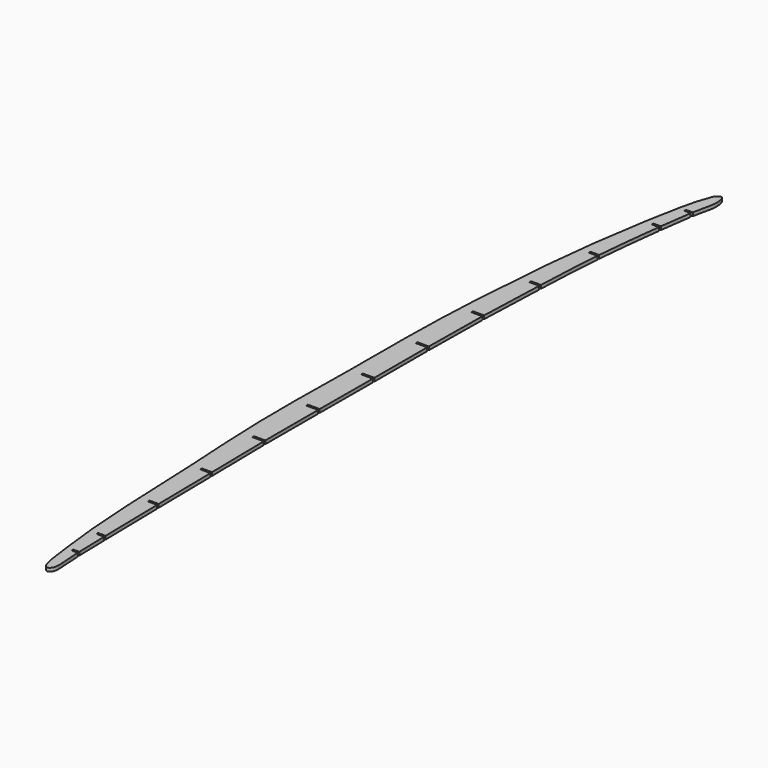
from build123d import *

# Parameters (mm, degrees)
F1_DEPTH = 10


# Not quite as in the source:
# - a feature names something its author has since deleted; it is built from what else it names


with BuildPart() as f1:
    # F0 (on Top) → F1 (new body)
    with BuildSketch(Plane.XY):
        with BuildLine():
            Line((-9.2522319783, 1105.5465694817), (-9.2522319783, 1108.5465694817))
            Line((-9.2522319783, 1108.5465694817), (-28.2522319783, 1108.5465694817))
            add(Edge.make_bspline(
                [(-28.2522319783, 1108.5465694817), (-34.1692287273, 1078.3481872981), (-40.0862254764, 1048.1498051145), (-46.885506853, 1008.5465694817)],
                knots=[0, 0, 0, 0, 0.0623728759, 0.0623728759, 0.0623728759, 0.0623728759], degree=3))
            Line((-46.885506853, 1008.5465694817), (-25.3817387583, 1008.5465694817))
            Line((-25.3817387583, 1008.5465694817), (-25.3817387583, 1011.5465694817))
            Line((-25.3817387583, 1011.5465694817), (-3.4951998214, 1011.5465694817))
            add(Edge.make_bspline(
                [(9.3214260817, 1105.5465694817), (5.2778951966, 1077.0910022719), (1.2125502532, 1048.3609188135), (-3.4951998214, 1011.5465694817)],
                knots=[0.0020582204, 0.0020582204, 0.0020582204, 0.0020582204, 0.0606128099, 0.0606128099, 0.0606128099, 0.0606128099], degree=3))
            Line((9.3214260817, 1105.5465694817), (-9.2522319783, 1105.5465694817))
        make_face()
        with BuildLine():
            Line((-28.2522319783, 1108.5465694817), (-9.2522319783, 1108.5465694817))
            Line((-9.2522319783, 1108.5465694817), (-9.2522319783, 1111.5465694817))
            Line((-9.2522319783, 1111.5465694817), (10.4483753261, 1111.5465694817))
            add(Edge.make_bspline(
                [(10.4483753261, 1111.5465694817), (14.2237569857, 1127.7176279013), (20.7843357368, 1156.0283342705), (24.50141426, 1181.1497468298), (21.913351831, 1202.3721726285), (17.2535020339, 1211.7645420112), (14.0231014783, 1212.5065694817)],
                knots=[0.0100141442, 0.0100141442, 0.0100141442, 0.0100141442, 0.1720322765, 0.2970501568, 0.4103591472, 0.4934759383, 0.4934759383, 0.4934759383, 0.4934759383], degree=3))
            add(Edge.make_bspline(
                [(14.0231014783, 1212.5065694817), (10.6916463361, 1213.2718093304), (0.9849483202, 1207.717065294), (-4.4652508998, 1194.4970040922), (-17.4495437423, 1158.8703779353), (-24.4328369098, 1126.3390394336), (-28.2522319783, 1108.5465694817)],
                knots=[0.4934759383, 0.4934759383, 0.4934759383, 0.4934759383, 0.5791928197, 0.6716390479, 0.8204084848, 1, 1, 1, 1], degree=3))
        make_face()
        with BuildLine():
            Line((-25.3817387583, 1008.5465694817), (-46.885506853, 1008.5465694817))
            add(Edge.make_bspline(
                [(-46.885506853, 1008.5465694817), (-56.4704307745, 952.7180223817), (-67.8086700034, 878.1997316325), (-76.2546409025, 808.5465694817)],
                knots=[0.0623728759, 0.0623728759, 0.0623728759, 0.0623728759, 0.1502997077, 0.1502997077, 0.1502997077, 0.1502997077], degree=3))
            Line((-76.2546409025, 808.5465694817), (-50.7523337375, 808.5465694817))
            Line((-50.7523337375, 808.5465694817), (-50.7523337375, 811.5465694817))
            Line((-50.7523337375, 811.5465694817), (-25.0042987138, 811.5465694817))
            add(Edge.make_bspline(
                [(-4.2590252459, 1005.5465694817), (-11.1919357354, 950.8419950912), (-19.4396527515, 879.0589079331), (-25.0042987138, 811.5465694817)],
                knots=[0.0637563334, 0.0637563334, 0.0637563334, 0.0637563334, 0.1487347177, 0.1487347177, 0.1487347177, 0.1487347177], degree=3))
            Line((-4.2590252459, 1005.5465694817), (-25.3817387583, 1005.5465694817))
            Line((-25.3817387583, 1005.5465694817), (-25.3817387583, 1008.5465694817))
        make_face()
        with BuildLine():
            Line((-50.7523337375, 808.5465694817), (-76.2546409025, 808.5465694817))
            add(Edge.make_bspline(
                [(-76.2546409025, 808.5465694817), (-84.6749646264, 739.1049172777), (-90.2205587707, 674.4988914733), (-95.4501271993, 608.5465694817)],
                knots=[0.1502997077, 0.1502997077, 0.1502997077, 0.1502997077, 0.2379595395, 0.2379595395, 0.2379595395, 0.2379595395], degree=3))
            Line((-95.4501271993, 608.5465694817), (-65.9492915816, 608.5465694817))
            Line((-65.9492915816, 608.5465694817), (-65.9492915816, 611.5465694817))
            Line((-65.9492915816, 611.5465694817), (-36.3208296657, 611.5465694817))
            add(Edge.make_bspline(
                [(-25.492600007, 805.5470480317), (-30.8991386303, 738.261256599), (-33.600522451, 675.484027067), (-36.3208296657, 611.5465694817)],
                knots=[0.1512568673, 0.1512568673, 0.1512568673, 0.1512568673, 0.2362855612, 0.2362855612, 0.2362855612, 0.2362855612], degree=3))
            Line((-25.492600007, 805.5470480317), (-50.8059161147, 805.5470480317))
            Line((-50.8059161147, 805.5470480317), (-50.7523337375, 808.5465694817))
        make_face()
        with BuildLine():
            Line((-65.9492915816, 608.5465694817), (-95.4501271993, 608.5465694817))
            add(Edge.make_bspline(
                [(-95.4501271993, 608.5465694817), (-100.6735657013, 542.6715546134), (-105.5817189232, 475.4533978756), (-108.8488180837, 408.5465694817)],
                knots=[0.2379595395, 0.2379595395, 0.2379595395, 0.2379595395, 0.3255166193, 0.3255166193, 0.3255166193, 0.3255166193], degree=3))
            Line((-108.8488180837, 408.5465694817), (-76.3366638949, 408.5465694817))
            Line((-76.3366638949, 408.5465694817), (-76.3366638949, 411.5465694817))
            Line((-76.3366638949, 411.5465694817), (-43.7472965242, 411.5465694817))
            add(Edge.make_bspline(
                [(-36.576081022, 605.5465694817), (-39.2965672487, 541.5968769288), (-42.0608997966, 476.4245488132), (-43.7472965243, 411.5465694817)],
                knots=[0.2389437345, 0.2389437345, 0.2389437345, 0.2389437345, 0.3238872962, 0.3238872962, 0.3238872962, 0.3238872962], degree=3))
            Line((-36.576081022, 605.5465694817), (-65.9492915816, 605.5465694817))
            Line((-65.9492915816, 605.5465694817), (-65.9492915816, 608.5465694817))
        make_face()
        with BuildLine():
            Line((-76.3366638949, 408.5465694817), (-108.8488180837, 408.5465694817))
            add(Edge.make_bspline(
                [(-108.8488180837, 408.5465694817), (-112.112873039, 341.7020832768), (-113.7389306982, 275.1683455095), (-114.3242902488, 208.5465694817)],
                knots=[0.3255166193, 0.3255166193, 0.3255166193, 0.3255166193, 0.4129921155, 0.4129921155, 0.4129921155, 0.4129921155], degree=3))
            Line((-114.3242902488, 208.5465694817), (-80.310060953, 208.5465694817))
            Line((-80.310060953, 208.5465694817), (-80.310060953, 211.5465694817))
            Line((-80.310060953, 211.5465694817), (-46.2853714025, 211.5465694817))
            add(Edge.make_bspline(
                [(-43.9001795453, 405.5465694817), (-45.519256644, 340.6971675299), (-46.0554016999, 276.1594412286), (-46.2853714025, 211.5465694817)],
                knots=[0.3265062426, 0.3265062426, 0.3265062426, 0.3265062426, 0.4114374445, 0.4114374445, 0.4114374445, 0.4114374445], degree=3))
            Line((-43.9001795453, 405.5465694817), (-76.3366638949, 405.5465694817))
            Line((-76.3366638949, 405.5465694817), (-76.3366638949, 408.5465694817))
        make_face()
        with BuildLine():
            Line((-80.310060953, 208.5465694817), (-114.3242902488, 208.5465694817))
            add(Edge.make_bspline(
                [(-114.3242902488, 208.5465694817), (-114.9095417049, 141.9370960513), (-114.4544793743, 75.2396168723), (-114.9729122534, 8.5465694817)],
                knots=[0.4129921155, 0.4129921155, 0.4129921155, 0.4129921155, 0.5004514582, 0.5004514582, 0.5004514582, 0.5004514582], degree=3))
            Line((-114.9729122534, 8.5465694817), (-80.772249135, 8.5465694817))
            Line((-80.772249135, 8.5465694817), (-80.772249135, 11.5465694817))
            Line((-80.772249135, 11.5465694817), (-46.5657327214, 11.5465694817))
            add(Edge.make_bspline(
                [(-46.3058677148, 205.5465694817), (-46.517541999, 140.9336478574), (-46.4426078998, 76.2408210046), (-46.5657327214, 11.5465694817)],
                knots=[0.4140662707, 0.4140662707, 0.4140662707, 0.4140662707, 0.4989910833, 0.4989910833, 0.4989910833, 0.4989910833], degree=3))
            Line((-46.3058677148, 205.5465694817), (-80.310060953, 205.5465694817))
            Line((-80.310060953, 205.5465694817), (-80.310060953, 208.5465694817))
        make_face()
        with BuildLine():
            Line((-80.772249135, 8.5465694817), (-114.9729122534, 8.5465694817))
            add(Edge.make_bspline(
                [(-114.9729122534, 8.5465694817), (-115.4913633728, -58.1488243975), (-116.9833782047, -124.8397861765), (-117.4326707445, -191.4534305183)],
                knots=[0.5004514582, 0.5004514582, 0.5004514582, 0.5004514582, 0.587913878, 0.587913878, 0.587913878, 0.587913878], degree=3))
            Line((-117.4326707445, -191.4534305183), (-82.4265356335, -191.4534305183))
            Line((-82.4265356335, -191.4534305183), (-82.4265356335, -188.4534305183))
            Line((-82.4265356335, -188.4534305183), (-47.4040323866, -188.4534305183))
            add(Edge.make_bspline(
                [(-46.5777314963, 5.5465694817), (-46.7134050172, -59.1479448978), (-47.0517150176, -123.8414273541), (-47.4040323866, -188.4534305183)],
                knots=[0.5016165032, 0.5016165032, 0.5016165032, 0.5016165032, 0.5865416442, 0.5865416442, 0.5865416442, 0.5865416442], degree=3))
            Line((-46.5777314963, 5.5465694817), (-80.772249135, 5.5465694817))
            Line((-80.772249135, 5.5465694817), (-80.772249135, 8.5465694817))
        make_face()
        with BuildLine():
            Line((-82.4265356335, -191.4534305183), (-117.4326707445, -191.4534305183))
            add(Edge.make_bspline(
                [(-117.4326707445, -191.4534305183), (-117.8819688578, -258.0679012195), (-117.2885188084, -324.6050525653), (-114.5979590791, -391.4534305183)],
                knots=[0.587913878, 0.587913878, 0.587913878, 0.587913878, 0.6753773828, 0.6753773828, 0.6753773828, 0.6753773828], degree=3))
            Line((-114.5979590791, -391.4534305183), (-81.0956338475, -391.4534305183))
            Line((-81.0956338475, -391.4534305183), (-81.0956338475, -388.4534305183))
            Line((-81.0956338475, -388.4534305183), (-47.6180785507, -388.4534305183))
            add(Edge.make_bspline(
                [(-47.4367827083, -194.4534305183), (-47.7896354912, -259.0626621028), (-48.1401096643, -323.5953829529), (-47.6180785507, -388.4534305183)],
                knots=[0.58917052, 0.58917052, 0.58917052, 0.58917052, 0.6740985981, 0.6740985981, 0.6740985981, 0.6740985981], degree=3))
            Line((-47.4367827083, -194.4534305183), (-82.4265356335, -194.4534305183))
            Line((-82.4265356335, -194.4534305183), (-82.4265356335, -191.4534305183))
        make_face()
        with BuildLine():
            Line((-81.0956338475, -391.4534305183), (-114.5979590791, -391.4534305183))
            add(Edge.make_bspline(
                [(-114.5979590791, -391.4534305183), (-111.9055675807, -458.347319741), (-107.1132099499, -525.5528594896), (-103.7767332928, -591.4534305183)],
                knots=[0.6753773828, 0.6753773828, 0.6753773828, 0.6753773828, 0.762900434, 0.762900434, 0.762900434, 0.762900434], degree=3))
            Line((-103.7767332928, -591.4534305183), (-74.0754674311, -591.4534305183))
            Line((-74.0754674311, -591.4534305183), (-74.0754674311, -588.4534305183))
            Line((-74.0754674311, -588.4534305183), (-44.426569062, -588.4534305183))
            add(Edge.make_bspline(
                [(-47.5672869388, -394.4534305183), (-46.9911709166, -459.3253273899), (-45.5476453008, -524.5049596078), (-44.426569062, -588.4534305183)],
                knots=[0.6767170821, 0.6767170821, 0.6767170821, 0.6767170821, 0.7616371329, 0.7616371329, 0.7616371329, 0.7616371329], degree=3))
            Line((-47.5672869388, -394.4534305183), (-81.0956338475, -394.4534305183))
            Line((-81.0956338475, -394.4534305183), (-81.0956338475, -391.4534305183))
        make_face()
        with BuildLine():
            Line((-74.0754674311, -591.4534305183), (-103.7767332928, -591.4534305183))
            add(Edge.make_bspline(
                [(-103.7767332928, -591.4534305183), (-100.4411938204, -657.3354907033), (-98.5607175504, -721.913315172), (-95.2888672995, -791.4534305183)],
                knots=[0.762900434, 0.762900434, 0.762900434, 0.762900434, 0.8503989007, 0.8503989007, 0.8503989007, 0.8503989007], degree=3))
            Line((-95.2888672995, -791.4534305183), (-68.2934120383, -791.4534305183))
            Line((-68.2934120383, -791.4534305183), (-68.2934120383, -788.4534305183))
            Line((-68.2934120383, -788.4534305183), (-41.3473226027, -788.4534305183))
            add(Edge.make_bspline(
                [(-44.3222964296, -594.4534305183), (-43.2214963704, -658.360909415), (-42.4517270587, -721.1021087734), (-41.3473226027, -788.4534305183)],
                knots=[0.7642946324, 0.7642946324, 0.7642946324, 0.7642946324, 0.8492622563, 0.8492622563, 0.8492622563, 0.8492622563], degree=3))
            Line((-44.3222964296, -594.4534305183), (-74.0754674311, -594.4534305183))
            Line((-74.0754674311, -594.4534305183), (-74.0754674311, -591.4534305183))
        make_face()
        with BuildLine():
            Line((-68.2934120383, -791.4534305183), (-95.2888672995, -791.4534305183))
            add(Edge.make_bspline(
                [(-95.2888672995, -791.4534305183), (-92.0149726534, -861.0369975725), (-87.3479647004, -935.5890587547), (-82.1628302646, -991.4534305183)],
                knots=[0.8503989007, 0.8503989007, 0.8503989007, 0.8503989007, 0.9379520403, 0.9379520403, 0.9379520403, 0.9379520403], degree=3))
            Line((-82.1628302646, -991.4534305183), (-59.7760454191, -991.4534305183))
            Line((-59.7760454191, -991.4534305183), (-59.7760454191, -988.4534305183))
            Line((-59.7760454191, -988.4534305183), (-37.4559647617, -988.4534305183))
            add(Edge.make_bspline(
                [(-41.2482418592, -794.4534305183), (-40.1266287573, -861.9004781348), (-38.6708390195, -933.7012026364), (-37.4559647617, -988.4534305183)],
                knots=[0.8517802395, 0.8517802395, 0.8517802395, 0.8517802395, 0.9365259774, 0.9365259774, 0.9365259774, 0.9365259774], degree=3))
            Line((-41.2482418592, -794.4534305183), (-68.2934120383, -794.4534305183))
            Line((-68.2934120383, -794.4534305183), (-68.2934120383, -791.4534305183))
        make_face()
        with BuildLine():
            Line((-59.7760454191, -991.4534305183), (-82.1628302646, -991.4534305183))
            add(Edge.make_bspline(
                [(-82.1628302646, -991.4534305183), (-78.4881817721, -1031.0439044063), (-74.5533092769, -1061.2486674623), (-70.6184367817, -1091.4534305183)],
                knots=[0.9379520403, 0.9379520403, 0.9379520403, 0.9379520403, 1, 1, 1, 1], degree=3))
            Line((-70.6184367817, -1091.4534305183), (-52.8165805825, -1091.4534305183))
            Line((-52.8165805825, -1091.4534305183), (-52.8165805825, -1088.4534305183))
            Line((-52.8165805825, -1088.4534305183), (-35.0888296498, -1088.4534305183))
            add(Edge.make_bspline(
                [(-37.322275987, -994.4534305183), (-36.4991726981, -1031.2396183628), (-35.7920332849, -1059.9830094592), (-35.0888296498, -1088.4534305183)],
                knots=[0.9396580371, 0.9396580371, 0.9396580371, 0.9396580371, 0.9979520124, 0.9979520124, 0.9979520124, 0.9979520124], degree=3))
            Line((-37.322275987, -994.4534305183), (-59.7760454191, -994.4534305183))
            Line((-59.7760454191, -994.4534305183), (-59.7760454191, -991.4534305183))
        make_face()
        with BuildLine():
            Line((-52.8165805825, -1091.4534305183), (-70.6184367817, -1091.4534305183))
            add(Edge.make_bspline(
                [(-70.6184367817, -1091.4534305183), (-67.9110233409, -1108.1005244006), (-63.3619889151, -1136.0712074231), (-62.8084472686, -1156.7636726537), (-56.9392429668, -1179.8854765827), (-52.0402683291, -1190.8912220635), (-43.8780764691, -1197.1956346468), (-35.6928205779, -1192.113746687), (-30.7731194715, -1181.9886543329), (-30.0475473892, -1169.6607279781), (-30.6576558665, -1159.033327889), (-30.985580365, -1153.3212537692)],
                knots=[0, 0, 0, 0, 0.1863834872, 0.3131641762, 0.4452842877, 0.5417120225, 0.6219151427, 0.7001120149, 0.7912063967, 0.8877764526, 1, 1, 1, 1], degree=3))
            add(Edge.make_bspline(
                [(-34.8233472068, -1094.4534305183), (-34.257564492, -1103.3212790556), (-33.0345610691, -1122.4536049764), (-31.700057419, -1142.5577425607), (-30.985580365, -1153.3212537692)],
                knots=[0.049793057, 0.049793057, 0.049793057, 0.049793057, 0.4912707377, 1, 1, 1, 1], degree=3))
            Line((-34.8233472068, -1094.4534305183), (-52.8165805825, -1094.4534305183))
            Line((-52.8165805825, -1094.4534305183), (-52.8165805825, -1091.4534305183))
        make_face()
    extrude(amount=F1_DEPTH)


solid = f1.part
